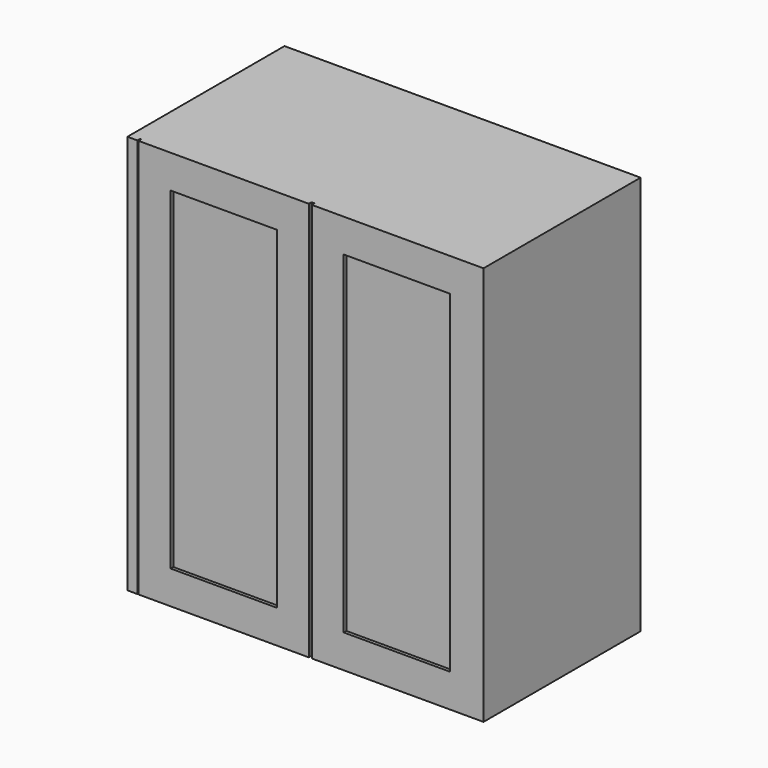
from build123d import *

# Parameters (mm, degrees)
F0_W     = 327.025
F0_H     = 762
F0_W_2   = 203.2
F0_H_2   = 635
F0_W_3   = 324.993
F0_W_4   = 3.175
F0_W_5   = 2.032
F1_DEPTH = 374.65
F2_DEPTH = 6.35
F3_W     = 368.3
F3_H     = 762
F3_W_2   = 247.65
F3_H_2   = 635
F3_W_3   = 6.35
F4_DEPTH = 19.05
F5_DEPTH = 12.7


# Not quite as in the source:
# - a feature names something its author has since deleted; it is built from what else it names


with BuildPart() as f1:
    # F0 (on Front) → F1 (new body)
    with BuildSketch(Plane.XZ):
        with Locations((394.5947425127, 381)):
            Rectangle(F0_W, F0_H)
        with Locations((393.0072425127, 381)):
            Rectangle(F0_W_2, F0_H_2, mode=Mode.SUBTRACT)
        with Locations((62.2357425127, 381)):
            Rectangle(F0_W_3, F0_H)
        with Locations((62.8072425127, 381)):
            Rectangle(F0_W_2, F0_H_2, mode=Mode.SUBTRACT)
        with Locations((62.8072425127, 381)):
            Rectangle(F0_W_2, F0_H_2)
        with Locations((393.0072425127, 381)):
            Rectangle(F0_W_2, F0_H_2)
        with Locations((226.3197425127, 381)):
            Rectangle(F0_W_4, F0_H)
        with Locations((229.4947425127, 381)):
            Rectangle(F0_W_4, F0_H)
        with Locations((-101.2767574873, 381)):
            Rectangle(F0_W_5, F0_H)
    extrude(amount=-F1_DEPTH)

    # F0 (on Front) → F2 (cut)
    with BuildSketch(Plane.XZ):
        with Locations((226.3197425127, 381)):
            Rectangle(F0_W_4, F0_H)
        with Locations((229.4947425127, 381)):
            Rectangle(F0_W_4, F0_H)
        with Locations((-101.2767574873, 381)):
            Rectangle(F0_W_5, F0_H)
        with Locations((62.8072425127, 381)):
            Rectangle(F0_W_2, F0_H_2)
        with Locations((393.0072425127, 381)):
            Rectangle(F0_W_2, F0_H_2)
    extrude(amount=-F2_DEPTH, mode=Mode.SUBTRACT)

    # F3 (on face) → F4 (join)
    with BuildSketch(Plane(origin=(-102.2927574873, 0, 0), x_dir=(0, -1, 0), z_dir=(-1, 0, 0))):
        with Locations((-190.5, 381)):
            Rectangle(F3_W, F3_H)
        with Locations((-187.325, 381)):
            Rectangle(F3_W_2, F3_H_2, mode=Mode.SUBTRACT)
        with Locations((-3.175, 381)):
            Rectangle(F3_W_3, F3_H)
    extrude(amount=F4_DEPTH)

    # F3 (on face) → F5 (join)
    with BuildSketch(Plane(origin=(-102.2927574873, 0, 0), x_dir=(0, -1, 0), z_dir=(-1, 0, 0))):
        with Locations((-187.325, 381)):
            Rectangle(F3_W_2, F3_H_2)
    extrude(amount=F5_DEPTH)


solid = f1.part
